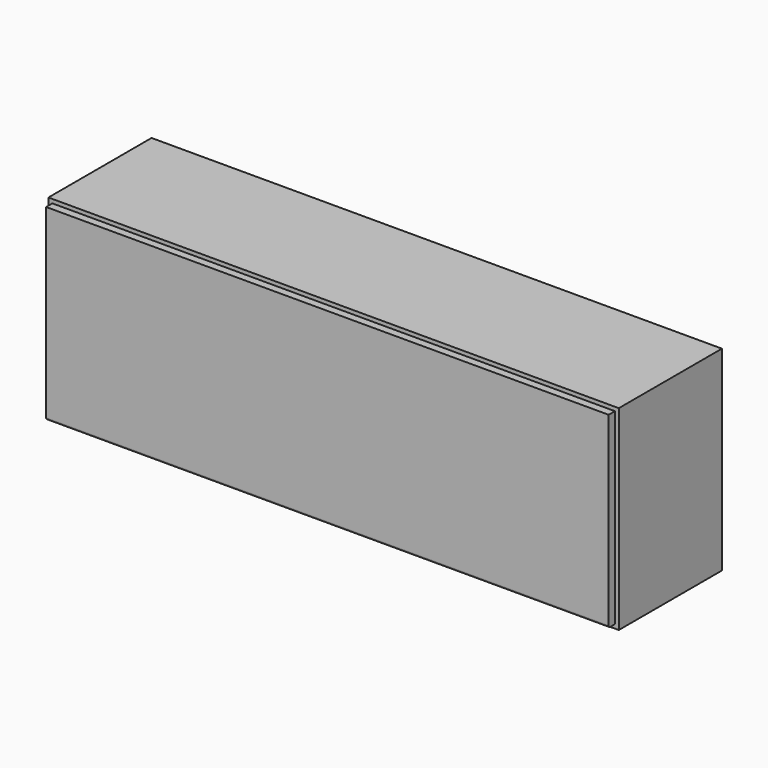
from build123d import *

# Parameters (mm, degrees)
F0_W     = 1460
F0_H     = 500
F1_DEPTH = 330
F2_T     = -25
F3_W     = 1440
F3_H     = 480
F4_DEPTH = 20
F5_R     = 5


# Not quite as in the source:
# - a feature names something its author has since deleted; it is built from what else it names


with BuildPart() as f1:
    # F0 (on Front) → F1 (new body)
    with BuildSketch(Plane.XZ):
        with Locations((0, 250)):
            Rectangle(F0_W, F0_H)
    extrude(amount=F1_DEPTH)

    # F2
    f2_openings = [f1.faces().sort_by_distance(p)[0] for p in [
        (0, -330, 250),
    ]]
    offset(amount=F2_T, openings=f2_openings)


with BuildPart() as f4:
    # F3 (on face) → F4 (new body)
    with BuildSketch(Plane.XZ.offset(330)):
        with Locations((0, 250)):
            Rectangle(F3_W, F3_H)
    extrude(amount=F4_DEPTH)

    # F5
    f5_edges = [f4.edges().sort_by_distance(p)[0] for p in [
        (0, -350, 10),
    ]]
    fillet(f5_edges, radius=F5_R)


solid = Compound([f1.part, f4.part])
